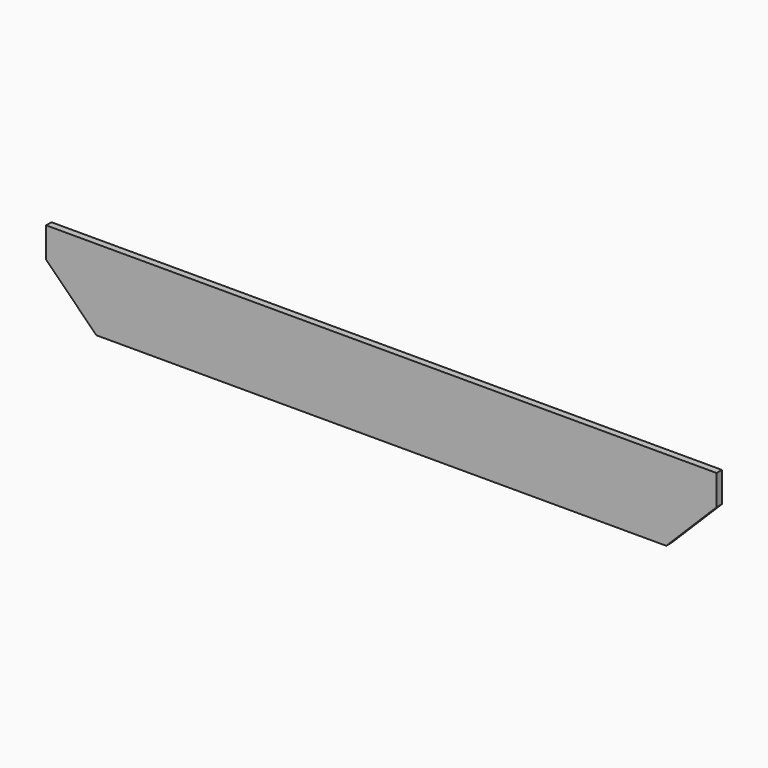
from build123d import *

# Parameters (mm, degrees)
F0_W     = 170
F0_H     = 15
F1_DEPTH = 2


# Not quite as in the source:
# - a feature names something its author has since deleted; it is built from what else it names


with BuildPart() as f1:
    # F0 (on Front) → F1 (new body)
    with BuildSketch(Plane.XZ):
        Rectangle(F0_W, F0_H)
        Polygon((-100, 7.5), (-85, -7.5), (-85, 7.5), align=None)
        Polygon((85, 7.5), (85, -7.5), (100, 7.5), align=None)
        Polygon((-85, 7.5), (85, 7.5), (100, 7.5), (100, 16.5), (-100, 16.5), (-100, 7.5), align=None)
    extrude(amount=F1_DEPTH)


solid = f1.part
